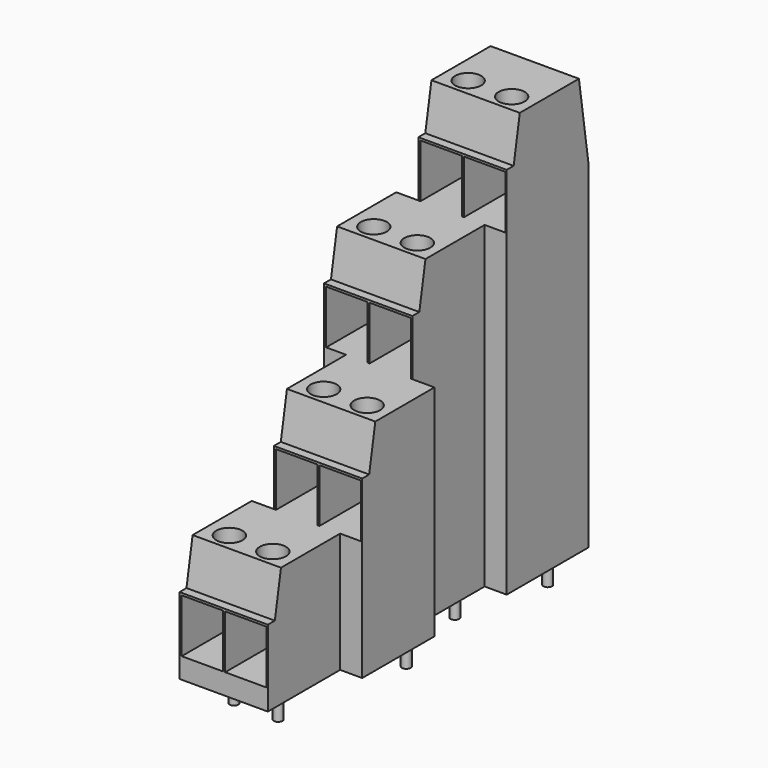
from build123d import *

# Parameters (mm, degrees)
F1_DEPTH  = 6.35
F3_DEPTH  = 2.54
F5_DEPTH  = 2.54
F6_W      = 4.75
F6_H      = 6.1595766147
F8_W      = 4.75
F8_H      = 6.1471766147
F7_W      = 4.75
F7_H      = 6.1471766147
F9_W      = 4.75
F9_H      = 6.1471766147
F10_DEPTH = 6
F11_R     = 1.5
F12_R     = 1.5
F13_R     = 1.5
F14_R     = 1.5
F15_DEPTH = 6
F16_R     = 0.5
F17_DEPTH = 3.5


# Not quite as in the source:
# - a feature names something its author has since deleted; it is built from what else it names


with BuildPart() as f1:
    # F0 (on Right) → F1 (new body, symmetric)
    with BuildSketch(Plane.YZ):
        Polygon((10.3821327425, 24.0797383321), (1.8821327425, 24.0797383321), (1, 19.0769149468), (0, 19.0769149468), (0, 12.6797383321), (-8.5, 12.6797383321), (-9.3821327425, 7.6769149468), (-10.3821327425, 7.6769149468), (-10.3821327425, 1.2797383321), (-18.8821327425, 1.2797383321), (-19.7642654851, -3.7230850532), (-20.7642654851, -3.7230850532), (-20.7642654851, -10.1202616679), (-29.2642654851, -10.1202616679), (-30.1463982276, -15.1230850532), (-31.1463982276, -15.1230850532), (-31.1463982276, -23.9202616679), (11.7536017724, -23.9202616679), (11.7536017724, 14.9208800867), align=None)
    extrude(amount=F1_DEPTH, both=True)

    # F2 (on face) → F3 (cut)
    with BuildSketch(Plane(origin=(-6.35, 0, 0), x_dir=(0, -1, 0), z_dir=(-1, 0, 0))):
        Polygon((-11.7536017724, -23.9202616679), (0, -23.9202616679), (0, 12.6797383321), (0, 19.0769149468), (-1, 19.0769149468), (-1.8821327425, 24.0797383321), (-10.3821327425, 24.0797383321), (-11.7536017724, 14.9208800867), align=None)
        Polygon((20.7642654851, -23.9202616679), (20.7642654851, -10.1202616679), (20.7642654851, -3.7230850532), (19.7642654851, -3.7230850532), (18.8821327425, 1.2797383321), (10.3821327425, 1.2797383321), (10.3821327425, -23.9202616679), align=None)
    extrude(amount=-F3_DEPTH, mode=Mode.SUBTRACT)

    # F4 (on face) → F5 (cut)
    with BuildSketch(Plane.YZ.offset(6.35)):
        Polygon((-20.7642654851, -23.9202616679), (-20.7642654851, -10.1202616679), (-29.2642654851, -10.1202616679), (-30.1463982276, -15.1230850532), (-31.1463982276, -15.1230850532), (-31.1463982276, -23.9202616679), align=None)
        Polygon((-10.3821327425, 1.2797383321), (-10.3821327425, -23.9202616679), (0, -23.9202616679), (0, 12.6797383321), (-8.5, 12.6797383321), (-9.3821327425, 7.6769149468), (-10.3821327425, 7.6769149468), align=None)
    extrude(amount=-F5_DEPTH, mode=Mode.SUBTRACT)

    # F6 (on face) + F8 (on face) + F7 (on face) + F9 (on face) → F10 (cut)
    with BuildSketch(Plane.XZ.offset(31.1463982276)):
        with Locations((-3.725, -18.4528733606)):
            Rectangle(F6_W, F6_H)
        with Locations((1.275, -18.4528733606)):
            Rectangle(F6_W, F6_H)
        with Locations((6.275, -18.4528733606)):
            Rectangle(F6_W, F6_H)
    with BuildSketch(Plane.XZ.offset(10.3821327425)):
        Polygon((-6.1, 7.4269149468), (-6.1, 1.2797383321), (-3.81, 1.2797383321), (-1.35, 1.2797383321), (-1.35, 7.4269149468), align=None)
        with Locations((1.275, 4.3533266394)):
            Rectangle(F8_W, F8_H)
        with Locations((6.275, 4.3533266394)):
            Rectangle(F8_W, F8_H)
    with BuildSketch(Plane.XZ.offset(20.7642654851)):
        with Locations((-1.185, -7.0466733606)):
            Rectangle(F7_W, F7_H)
        Polygon((1.44, -3.9730850532), (1.44, -10.1202616679), (3.81, -10.1202616679), (6.19, -10.1202616679), (6.19, -3.9730850532), align=None)
        with Locations((8.815, -7.0466733606)):
            Rectangle(F7_W, F7_H)
    with BuildSketch(Plane.XZ):
        with Locations((-1.185, 15.7533266394)):
            Rectangle(F9_W, F9_H)
        Polygon((1.44, 18.8269149468), (1.44, 12.6797383321), (3.81, 12.6797383321), (6.19, 12.6797383321), (6.19, 18.8269149468), align=None)
        with Locations((8.815, 15.7533266394)):
            Rectangle(F9_W, F9_H)
    extrude(amount=-F10_DEPTH, mode=Mode.SUBTRACT)

    # F11 (on face) + F12 (on face) + F13 (on face) + F14 (on face) → F15 (cut)
    with BuildSketch(Plane.XY.offset(-10.1202616679)):
        with Locations((-3.725, -27.2642654851)):
            Circle(F11_R)
        with Locations((1.275, -27.2642654851)):
            Circle(F11_R)
        with Locations((6.275, -27.2642654851)):
            Circle(F11_R)
    with BuildSketch(Plane.XY.offset(1.2797383321)):
        with Locations((-1.185, -16.8821327425)):
            Circle(F12_R)
        with Locations((3.815, -16.8821327425)):
            Circle(F12_R)
        with Locations((8.815, -16.8821327425)):
            Circle(F12_R)
    with BuildSketch(Plane.XY.offset(12.6797383321)):
        with Locations((-3.725, -6.5)):
            Circle(F13_R)
        with Locations((1.275, -6.5)):
            Circle(F13_R)
        with Locations((6.275, -6.5)):
            Circle(F13_R)
    with BuildSketch(Plane.XY.offset(24.0797383321)):
        with Locations((-1.185, 3.8821327425)):
            Circle(F14_R)
        with Locations((3.815, 3.8821327425)):
            Circle(F14_R)
        with Locations((8.815, 3.8821327425)):
            Circle(F14_R)
    extrude(amount=-F15_DEPTH, mode=Mode.SUBTRACT)

    # F16 (on face) → F17 (join)
    with BuildSketch(Plane(origin=(0, 0, -23.9202616679), x_dir=(1, 0, 0), z_dir=(0, 0, -1))):
        with Locations((1.27, 26.4963982276)):
            Circle(F16_R)
        with Locations((-3.81, 26.4963982276)):
            Circle(F16_R)
        with Locations((3.81, 11.2563982276)):
            Circle(F16_R)
        with Locations((-1.27, 11.2563982276)):
            Circle(F16_R)
        with Locations((-3.81, 1.0963982276)):
            Circle(F16_R)
        with Locations((1.27, 1.0963982276)):
            Circle(F16_R)
        with Locations((3.81, -9.0636017724)):
            Circle(F16_R)
        with Locations((-1.27, -9.0636017724)):
            Circle(F16_R)
    extrude(amount=F17_DEPTH)


solid = f1.part
